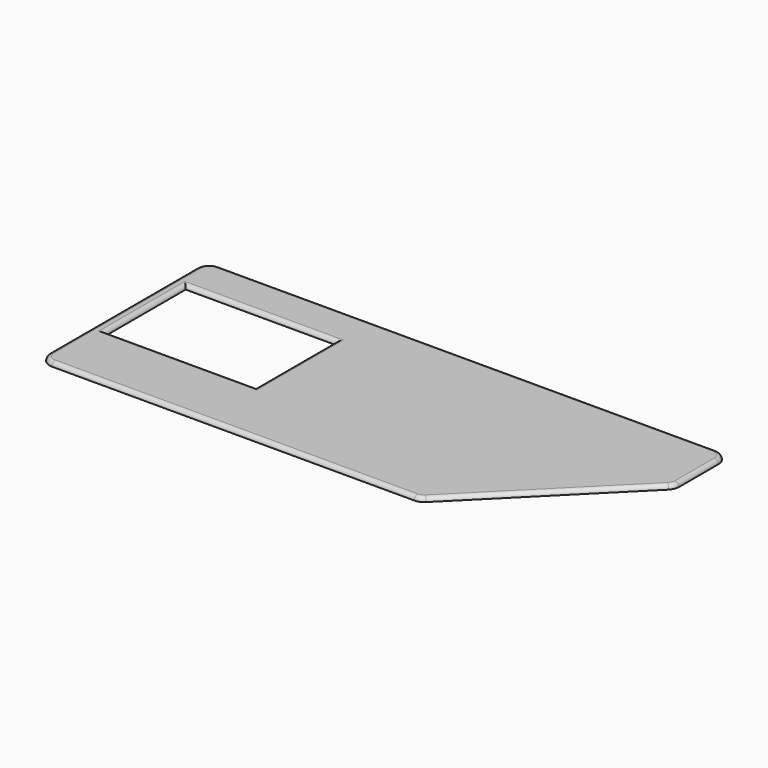
from build123d import *

# Parameters (mm, degrees)
F1_DEPTH = 1
F2_W     = 36
F2_H     = 24
F3_DEPTH = 25
F4_R     = 3
F5_R     = 0.99999


# Not quite as in the source:
# - a fillet or chamfer is up to 0.001 mm smaller than in the source, because OpenCascade refuses the exact size


with BuildPart() as f1:
    # F0 (on Top) → F1 (new body)
    with BuildSketch(Plane.XY):
        Polygon((62.5, 9), (62.5, 25), (-62.5, 25), (-62.5, -25), (28.5, -25), align=None)
    extrude(amount=F1_DEPTH)

    # F2 (on face) → F3 (cut)
    with BuildSketch(Plane.XY.offset(1)):
        with Locations((-41.5, 3)):
            Rectangle(F2_W, F2_H)
    extrude(amount=-F3_DEPTH, mode=Mode.SUBTRACT)

    # F4
    f4_edges = [f1.edges().sort_by_distance(p)[0] for p in [
        (-62.5, 25, 0.5),
        (-62.5, -25, 0.5),
        (62.5, 25, 0.5),
        (28.5, -25, 0.5),
        (62.5, 9, 0.5),
    ]]
    fillet(f4_edges, radius=F4_R)

    # F5 (radius 1 in the source; OpenCascade refuses exactly that, so slightly less here)
    f5_edges = [f1.edges().sort_by_distance(p)[0] for p in [
        (62.5, 16.12132, 1),
        (62.271639, 9.09459, 1),
        (61.62132, 24.12132, 1),
        (45.5, -8, 1),
        (0, 25, 1),
        (28.40541, -24.771639, 1),
        (-61.62132, 24.12132, 1),
        (-16.12132, -25, 1),
        (-62.5, 0, 1),
        (-61.62132, -24.12132, 1),
        (-23.5, 3, 1),
        (-41.5, 15, 1),
        (-59.5, 3, 1),
        (-41.5, -9, 1),
    ]]
    fillet(f5_edges, radius=F5_R)


solid = f1.part
